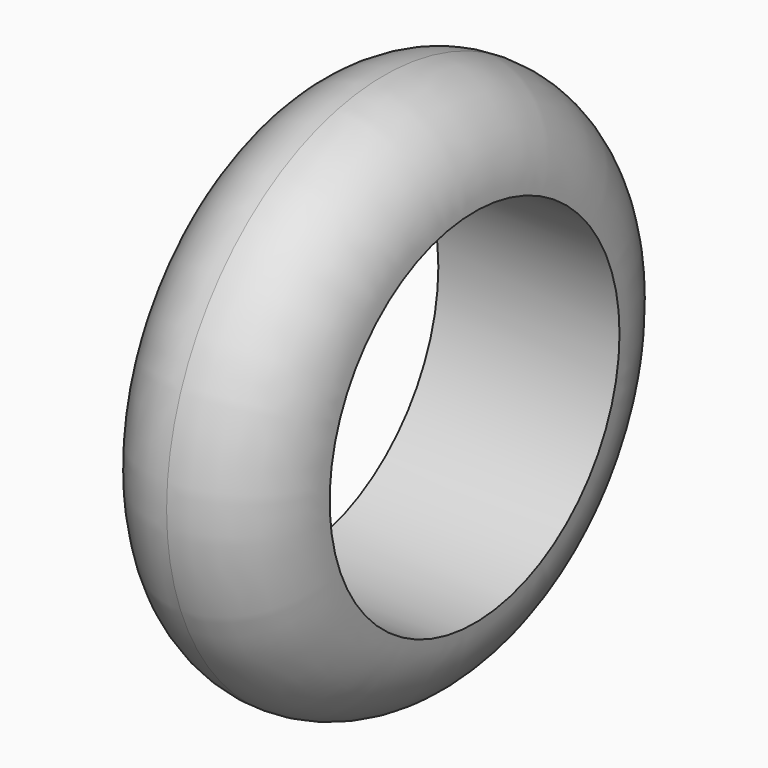
from build123d import *

# Parameters (mm, degrees)
F0_R     = 19.05
F0_R_2   = 12.7
F1_DEPTH = 12.7
F2_R     = 6.34999


# Not quite as in the source:
# - a fillet or chamfer is up to 0.001 mm smaller than in the source, because OpenCascade refuses the exact size


with BuildPart() as f1:
    # F0 (on Right) → F1 (new body)
    with BuildSketch(Plane.YZ):
        Circle(F0_R)
        Circle(F0_R_2, mode=Mode.SUBTRACT)
    extrude(amount=F1_DEPTH)

    # F2 (radius 6.35 in the source; OpenCascade refuses exactly that, so slightly less here)
    f2_edges = [f1.edges().sort_by_distance(p)[0] for p in [
        (12.7, -19.05, 0),
        (0, -19.05, 0),
    ]]
    fillet(f2_edges, radius=F2_R)


solid = f1.part
